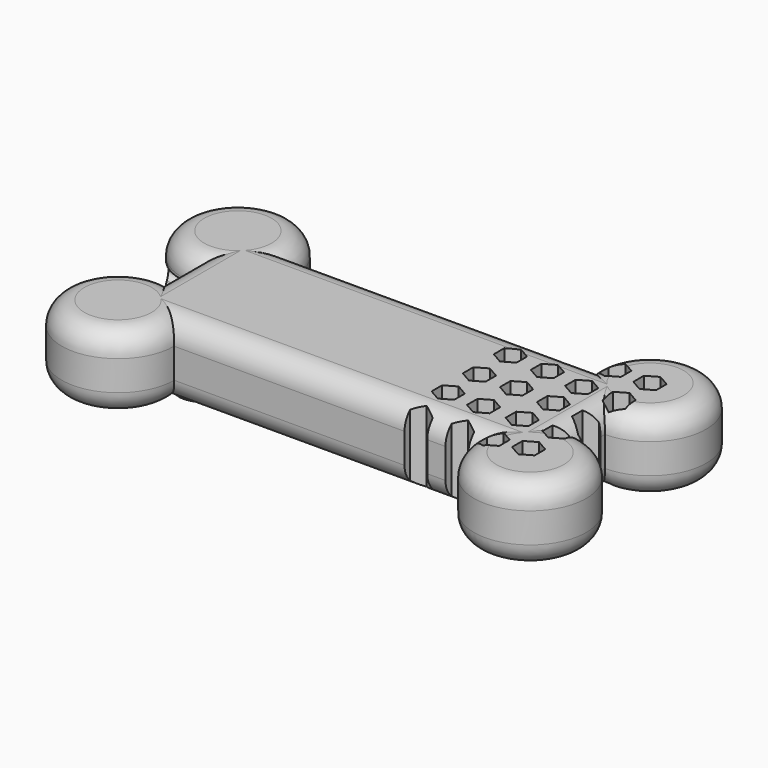
from build123d import *

# Parameters (mm, degrees)
F1_DEPTH     = 12.7
F2_R         = 7.62
F4_DEPTH     = 105.156
F4_TAPER     = 3
F6_DEPTH     = 41.402
F7_TEXT_SIZE = 22.168095
F8_DEPTH     = 2.54


# Not quite as in the source:
# - Text() gives the source's letters only with a copy of the font that has no kerning and outlines rounded to 1/6400 em; it was checked with that copy


with BuildPart() as f1:
    # F0 (on Top) → F1 (new body, symmetric)
    with BuildSketch(Plane.XY):
        with BuildLine():
            Line((50.8, 25.4), (-50.8, 25.4))
            ThreePointArc((-50.8, 25.4), (-83.320384, 38.870384), (-69.85, 6.35))
            Line((-69.85, 6.35), (-69.85, -6.35))
            ThreePointArc((-69.85, -6.35), (-83.320384, -38.870384), (-50.8, -25.4))
            Line((-50.8, -25.4), (50.8, -25.4))
            ThreePointArc((50.8, -25.4), (83.320384, -38.870384), (69.85, -6.35))
            Line((69.85, -6.35), (69.85, 6.35))
            ThreePointArc((69.85, 6.35), (83.320384, 38.870384), (50.8, 25.4))
        make_face()
    extrude(amount=F1_DEPTH, both=True)

    # F2
    f2_edges = [f1.edges().sort_by_distance(p)[0] for p in [
        (-83.320384, -38.870384, 12.7),
        (-69.85, 0, 12.7),
        (-83.320384, 38.870384, 12.7),
        (-83.320384, -38.870384, -12.7),
        (-69.85, 0, -12.7),
        (-83.320384, 38.870384, -12.7),
        (0, -25.4, 12.7),
        (0, 25.4, 12.7),
        (83.320384, -38.870384, 12.7),
        (69.85, 0, 12.7),
        (83.320384, 38.870384, 12.7),
        (69.85, 0, -12.7),
        (83.320384, 38.870384, -12.7),
        (83.320384, -38.870384, -12.7),
        (0, -25.4, -12.7),
        (0, 25.4, -12.7),
    ]]
    fillet(f2_edges, radius=F2_R)

    # F3 (on Right) → F4 (cut)
    with BuildSketch(Plane.YZ):
        with BuildLine():
            ThreePointArc((22.225, 1.905), (20.365128, 6.395128), (15.875, 8.255))
            Line((15.875, 8.255), (-15.875, 8.255))
            ThreePointArc((-15.875, 8.255), (-20.365128, 6.395128), (-22.225, 1.905))
            Line((-22.225, 1.905), (-22.225, -1.905))
            ThreePointArc((-22.225, -1.905), (-20.365128, -6.395128), (-15.875, -8.255))
            Line((-15.875, -8.255), (15.875, -8.255))
            ThreePointArc((15.875, -8.255), (20.365128, -6.395128), (22.225, -1.905))
            Line((22.225, -1.905), (22.225, 1.905))
        make_face()
    extrude(amount=-F4_DEPTH, taper=F4_TAPER, mode=Mode.SUBTRACT)

    # F5 (on face) → F6 (cut)
    with BuildSketch(Plane.XY.offset(12.7)):
        Polygon((73.699483, 23.1775), (73.699483, 27.6225), (69.85, 29.845), (66.000517, 27.6225), (66.000517, 23.1775), (69.85, 20.955), align=None)
        Polygon((73.073776, 10.884324), (73.073776, 15.329324), (69.224293, 17.551824), (65.37481, 15.329324), (65.37481, 10.884324), (69.224293, 8.661824), align=None)
        Polygon((72.746137, -1.628477), (72.746137, 2.816523), (68.896654, 5.039023), (65.047171, 2.816523), (65.047171, -1.628477), (68.896654, -3.850977), align=None)
        Polygon((72.166839, -13.640483), (72.166839, -9.195483), (68.317356, -6.972983), (64.467873, -9.195483), (64.467873, -13.640483), (68.317356, -15.862983), align=None)
        Polygon((71.971075, -26.071457), (71.971075, -21.626457), (68.121592, -19.403957), (64.272109, -21.626457), (64.272109, -26.071457), (68.121592, -28.293957), align=None)
        Polygon((61.668632, 23.321337), (61.668632, 27.766337), (57.819149, 29.988837), (53.969666, 27.766337), (53.969666, 23.321337), (57.819149, 21.098837), align=None)
        Polygon((61.028188, 10.085483), (61.028188, 14.530483), (57.178705, 16.752983), (53.329222, 14.530483), (53.329222, 10.085483), (57.178705, 7.862983), align=None)
        Polygon((61.028188, -1.869478), (61.028188, 2.575522), (57.178705, 4.798022), (53.329222, 2.575522), (53.329222, -1.869478), (57.178705, -4.091978), align=None)
        Polygon((60.174262, -14.037922), (60.174262, -9.592922), (56.324779, -7.370422), (52.475296, -9.592922), (52.475296, -14.037922), (56.324779, -16.260422), align=None)
        Polygon((61.241669, -27.700736), (61.241669, -23.255736), (57.392186, -21.033236), (53.542703, -23.255736), (53.542703, -27.700736), (57.392186, -29.923236), align=None)
        Polygon((48.859743, -27.273774), (48.859743, -22.828774), (45.01026, -20.606274), (41.160777, -22.828774), (41.160777, -27.273774), (45.01026, -29.496274), align=None)
        Polygon((47.578854, -14.678367), (47.578854, -10.233367), (43.729371, -8.010867), (39.879888, -10.233367), (39.879888, -14.678367), (43.729371, -16.900867), align=None)
        Polygon((48.005817, -1.229034), (48.005817, 3.215966), (44.156334, 5.438466), (40.306851, 3.215966), (40.306851, -1.229034), (44.156334, -3.451534), align=None)
        Polygon((48.219298, 11.579854), (48.219298, 16.024854), (44.369816, 18.247354), (40.520333, 16.024854), (40.520333, 11.579854), (44.369816, 9.357354), align=None)
        Polygon((47.365373, 23.321337), (47.365373, 27.766337), (43.51589, 29.988837), (39.666407, 27.766337), (39.666407, 23.321337), (43.51589, 21.098837), align=None)
        Polygon((36.050858, 24.388742), (36.050858, 28.833742), (32.201375, 31.056242), (28.351892, 28.833742), (28.351892, 24.388742), (32.201375, 22.166242), align=None)
        Polygon((34.983448, 12.433778), (34.983448, 16.878778), (31.133965, 19.101278), (27.284482, 16.878778), (27.284482, 12.433778), (31.133965, 10.211278), align=None)
        Polygon((35.410413, -1.229034), (35.410413, 3.215966), (31.56093, 5.438466), (27.711447, 3.215966), (27.711447, -1.229034), (31.56093, -3.451534), align=None)
        Polygon((35.410413, -14.464885), (35.410413, -10.019885), (31.56093, -7.797385), (27.711447, -10.019885), (27.711447, -14.464885), (31.56093, -16.687385), align=None)
        Polygon((34.983448, -27.487255), (34.983448, -23.042255), (31.133965, -20.819755), (27.284482, -23.042255), (27.284482, -27.487255), (31.133965, -29.709755), align=None)
    extrude(amount=-F6_DEPTH, mode=Mode.SUBTRACT)

    # F7 (on face) → F8 (join)
    with BuildSketch(Plane(origin=(0, 0, -12.7), x_dir=(1, 0, 0), z_dir=(0, 0, -1))):
        with Locations((-62.23, 0.919552)):
            Text('Sanso', F7_TEXT_SIZE, font='Open Sans', font_style=FontStyle.BOLDITALIC, text_align=(TextAlign.LEFT, TextAlign.BOTTOM))
    extrude(amount=F8_DEPTH)


solid = f1.part
